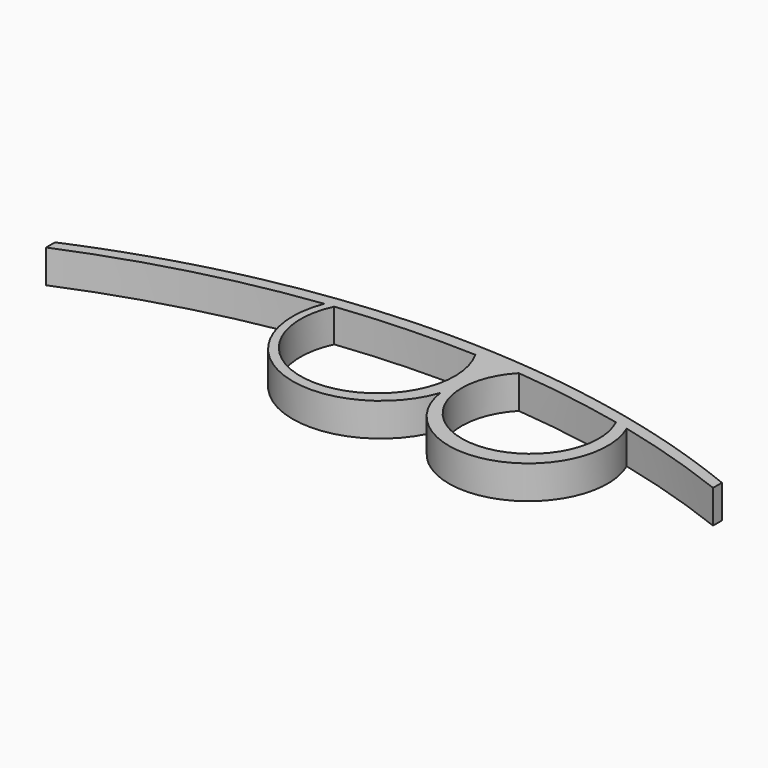
from build123d import *

# Parameters (mm, degrees)
F1_DEPTH = 7.62


# Not quite as in the source:
# - a feature names something its author has since deleted; it is built from what else it names


with BuildPart() as f1:
    # F0 (on Top) → F1 (new body)
    with BuildSketch(Plane.XY):
        with BuildLine():
            ThreePointArc((28.0726799719, -12.1853696085), (41.4217161306, -15.8764714027), (54.48557809, -20.4760919879))
            Line((54.48557809, -20.4760919879), (54.48557809, -17.9360919879))
            ThreePointArc((54.48557809, -17.9360919879), (51.4967288592, -16.763821011), (48.4891792987, -15.6403956202))
            ThreePointArc((48.4891792987, -15.6403956202), (44.8602983758, -14.3584600038), (41.2070755106, -13.1476345109))
            ThreePointArc((41.2070755106, -13.1476345109), (38.6048957608, -12.3330871208), (35.9916952796, -11.5546205858))
            ThreePointArc((35.9916952796, -11.5546205858), (31.733320464, -10.3696867585), (27.4494413676, -9.2805567694))
            ThreePointArc((27.4494413676, -9.2805567694), (23.9583783923, -8.4680969379), (20.4531163964, -7.7192645032))
            ThreePointArc((20.4531163964, -7.7192645032), (16.632517094, -6.9785468001), (12.7980359257, -6.3134183048))
            ThreePointArc((12.7980359257, -6.3134183048), (8.7921771864, -5.7014539178), (4.7745823593, -5.1719858311))
            ThreePointArc((4.7745823593, -5.1719858311), (2.3888765712, -4.897241097), (0, -4.6515878779))
            ThreePointArc((0, -4.6515878779), (-3.408711726, -4.3518848821), (-6.8221133026, -4.111412028))
            ThreePointArc((-6.8221133026, -4.111412028), (-10.4071482604, -3.922869598), (-13.9950228451, -3.7996630199))
            ThreePointArc((-13.9950228451, -3.7996630199), (-17.6605592517, -3.7413156735), (-21.3265467845, -3.7511630261))
            ThreePointArc((-21.3265467845, -3.7511630261), (-24.644831847, -3.8188928365), (-27.9615056934, -3.9424957507))
            ThreePointArc((-27.9615056934, -3.9424957507), (-43.2450696176, -5.2385218831), (-58.3815462887, -7.7192645032))
            ThreePointArc((-58.3815462887, -7.7192645032), (-63.1505292395, -8.7544721801), (-67.8924174044, -9.907446573))
            ThreePointArc((-67.8924174044, -9.907446573), (-73.5380139988, -11.4440807397), (-79.1355054029, -13.1476345109))
            ThreePointArc((-79.1355054029, -13.1476345109), (-81.4068857464, -13.8911431732), (-83.6690823894, -14.6621426181))
            ThreePointArc((-83.6690823894, -14.6621426181), (-86.1587803012, -15.5463139993), (-88.6364011403, -16.4637831816))
            ThreePointArc((-88.6364011403, -16.4637831816), (-89.8911745679, -16.9429103569), (-91.1426533968, -17.430578221))
            ThreePointArc((-91.1426533968, -17.430578221), (-92.6613427932, -18.0356268436), (-94.1749608987, -18.6532525791))
            ThreePointArc((-94.1749608987, -18.6532525791), (-95.4778611275, -19.1966804672), (-96.7768352111, -19.7494274307))
            Line((-96.7768352111, -19.7494274307), (-96.7768352111, -22.2894274307))
            ThreePointArc((-96.7768352111, -22.2894274307), (-71.0235394951, -13.4887335549), (-44.319003481, -8.239713722))
            ThreePointArc((-44.319003481, -8.239713722), (-43.2806848499, -8.1104188526), (-42.2417086499, -7.9865188972))
            ThreePointArc((-42.2417086499, -7.9865188972), (-26.5950201746, -6.7772498749), (-10.9016764341, -6.7896617958))
            ThreePointArc((-10.9016764341, -6.7896617958), (-6.4890042329, -7.0136625153), (-2.0823062052, -7.3343878974))
            ThreePointArc((-2.0823062052, -7.3343878974), (-1.2360355683, -7.4071155247), (-0.3900791081, -7.4834107816))
            ThreePointArc((-0.3900791081, -7.4834107816), (12.3943473899, -9.0773217505), (25.050742044, -11.4851812603))
            ThreePointArc((25.050742044, -11.4851812603), (26.5630587768, -11.8294586082), (28.0726799719, -12.1853696085))
        make_face()
        with BuildLine():
            ThreePointArc((-44.319003481, -8.239713722), (-32.5703828211, -34.4389737288), (-6.5546215011, -22.2894274307))
            ThreePointArc((-6.5546215011, -22.2894274307), (-6.0039890378, -14.307850149), (-2.0823062052, -7.3343878974))
            ThreePointArc((-2.0823062052, -7.3343878974), (-6.4890042329, -7.0136625153), (-10.9016764341, -6.7896617958))
            ThreePointArc((-10.9016764341, -6.7896617958), (-25.5859305121, -33.2005400837), (-42.2417086499, -7.9865188972))
            ThreePointArc((-42.2417086499, -7.9865188972), (-43.2806848499, -8.1104188526), (-44.319003481, -8.239713722))
        make_face()
        with BuildLine():
            ThreePointArc((-6.5546215011, -22.2894274307), (16.5208344464, -36.9835014795), (28.0726799719, -12.1853696085))
            ThreePointArc((28.0726799719, -12.1853696085), (26.5630587768, -11.8294586082), (25.050742044, -11.4851812603))
            ThreePointArc((25.050742044, -11.4851812603), (8.5004214133, -33.8325331942), (-0.3900791081, -7.4834107816))
            ThreePointArc((-0.3900791081, -7.4834107816), (-1.2360355683, -7.4071155247), (-2.0823062052, -7.3343878974))
            ThreePointArc((-2.0823062052, -7.3343878974), (-6.0039890378, -14.307850149), (-6.5546215011, -22.2894274307))
        make_face()
    extrude(amount=F1_DEPTH)


solid = f1.part
